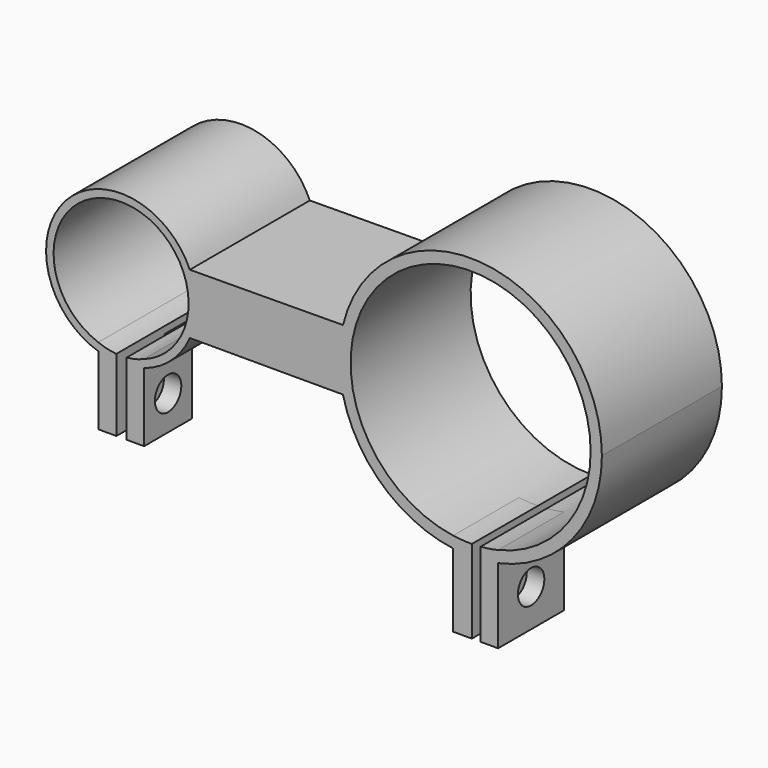
from build123d import *

# Parameters (mm, degrees)
F0_R      = 12.7
F0_R_2    = 11.43
F1_DEPTH  = 25.4
F3_R      = 20.32
F4_DEPTH  = 25.4
F5_W      = 3.0645749275
F5_H      = 25.4
F6_DEPTH  = 10.16
F8_DEPTH  = 30.226
F9_DEPTH  = 25.4
F10_R     = 2.794
F11_DEPTH = 25.4
F13_W     = 3.175
F13_H     = 35.56
F14_DEPTH = 13.97
F15_R     = 2.794
F16_DEPTH = 25.4
F18_DEPTH = 30.734
F20_DEPTH = 40.64
F22_DEPTH = 25.4


with BuildPart() as f1:
    # F0 (on Front) → F1 (new body)
    with BuildSketch(Plane.XZ):
        Circle(F0_R)
        Circle(F0_R_2, mode=Mode.SUBTRACT)
    extrude(amount=F1_DEPTH)

    # F5 (on offset) → F6 (join)
    with BuildSketch(Plane.XZ.offset(25.4)):
        with Locations((-2.327306883, -11.0291545425)):
            Rectangle(F5_W, F5_H)
        Polygon((3.894138498, 1.6708454575), (0.9391864802, 1.6708454575), (0.9391864802, -23.7291545425), (3.894138498, -23.7291545425), (3.894138498, -11.0291545425), align=None)
    extrude(amount=-F6_DEPTH)

    # F7 (on face) → F8 (cut)
    with BuildSketch(Plane.XZ.offset(25.4)):
        Polygon((-3.8595943467, 6.5400209701), (-3.8595943467, -10.7586445001), (-0.7950194192, -10.7537217399), (0.9391864802, -10.7509360094), (3.894138498, -10.7461893413), (3.894138498, 6.8227690223), align=None)
        Polygon((0.9391864802, -10.7509360094), (-0.7950194192, -10.7537217399), (-0.7950194192, -12.6750914838), (0.9391864802, -12.6652251759), (0.9391864802, -11.3913488558), align=None)
    extrude(amount=-F8_DEPTH, mode=Mode.SUBTRACT)

    # F7 (on face) → F9 (cut)
    with BuildSketch(Plane.XZ.offset(25.4)):
        Polygon((-3.8595943467, 6.5400209701), (-3.8595943467, -10.7586445001), (-0.7950194192, -10.7537217399), (0.9391864802, -10.7509360094), (3.894138498, -10.7461893413), (3.894138498, 6.8227690223), align=None)
        Polygon((0.9391864802, -10.7509360094), (-0.7950194192, -10.7537217399), (-0.7950194192, -12.6750914838), (0.9391864802, -12.6652251759), (0.9391864802, -11.3913488558), align=None)
    extrude(amount=-F9_DEPTH, mode=Mode.SUBTRACT)

    # F10 (on face) → F11 (cut)
    with BuildSketch(Plane(origin=(-3.8595943467, 0, 0), x_dir=(0, -1, 0), z_dir=(-1, 0, 0))):
        with Locations((20.32, -17.914237003)):
            Circle(F10_R)
    extrude(amount=-F11_DEPTH, mode=Mode.SUBTRACT)


with BuildPart() as f4:
    # F3 (on offset) → F4 (new body)
    with BuildSketch(Plane.XZ.offset(25.4)):
        with BuildLine():
            Line((37.5699403561, 5.2842361421), (10.6034887032, 5.0843427817))
            ThreePointArc((10.6034887032, 5.0843427817), (11.5328465432, 2.6263680661), (11.8205691299, 0.0143647333))
            Line((11.8205691299, 0.0143647333), (36.950101903, 0.0449029444))
            ThreePointArc((36.950101903, 0.0449029444), (37.1040026209, 2.6830272873), (37.5699403561, 5.2842361421))
        make_face()
        with BuildLine():
            ThreePointArc((81.4000854922, 0.0719114545), (61.799611578, 22.1414036966), (37.5699403561, 5.2842361421))
            Line((37.5699403561, 5.2842361421), (38.7200076161, 5.2927612092))
            ThreePointArc((38.7200076161, 5.2927612092), (37.3247254516, 0.1119146147), (38.6803581082, -5.079447813))
            Line((38.6803581082, -5.079447813), (37.5553231739, -5.079447813))
            ThreePointArc((37.5553231739, -5.079447813), (61.7684816706, -22.0012605256), (81.4000854922, 0.0719114545))
        make_face()
        with Locations((59.1750854922, 0.0719114545)):
            Circle(F3_R, mode=Mode.SUBTRACT)
        with BuildLine():
            Line((38.7200076161, 5.2927612092), (37.5699403561, 5.2842361421))
            ThreePointArc((37.5699403561, 5.2842361421), (37.1040026209, 2.6830272873), (36.950101903, 0.0449029444))
            ThreePointArc((36.950101903, 0.0449029444), (37.1034933748, -2.5348962497), (37.5553231739, -5.079447813))
            Line((37.5553231739, -5.079447813), (38.6803581082, -5.079447813))
            ThreePointArc((38.6803581082, -5.079447813), (37.3247254516, 0.1119146147), (38.7200076161, 5.2927612092))
        make_face()
        with BuildLine():
            Line((36.950101903, 0.0449029444), (11.8205691299, 0.0143647333))
            ThreePointArc((11.8205691299, 0.0143647333), (11.4383828548, -2.6236056978), (10.4021426077, -5.079447813))
            Line((10.4021426077, -5.079447813), (37.5553231739, -5.079447813))
            ThreePointArc((37.5553231739, -5.079447813), (37.1034933748, -2.5348962497), (36.950101903, 0.0449029444))
        make_face()
    extrude(amount=-F4_DEPTH)


with BuildPart() as f1_1:
    add(f1.part)

    # F12: union F4
    add(f4.part)

    # F13 (on face) → F14 (join)
    with BuildSketch(Plane.XZ.offset(25.4)):
        Polygon((63.8311807601, 1.2001052282), (60.8582296082, 1.2001052282), (60.8582296082, -34.3598947718), (63.8311807601, -34.3598947718), (63.8311807601, -21.6598947718), align=None)
        with Locations((57.7986807601, -16.5798947718)):
            Rectangle(F13_W, F13_H)
    extrude(amount=-F14_DEPTH)

    # F15 (on face) → F16 (cut)
    with BuildSketch(Plane.YZ.offset(63.8311807601)):
        with Locations((-18.415, -28.0098947718)):
            Circle(F15_R)
    extrude(amount=-F16_DEPTH, mode=Mode.SUBTRACT)

    # F17 (on face) → F18 (cut)
    with BuildSketch(Plane.XZ.offset(25.4)):
        with BuildLine():
            ThreePointArc((63.8311807601, -19.7074509431), (58.3136851955, 20.3736451127), (56.2111807601, -20.0307666939))
            Line((56.2111807601, -20.0307666939), (56.2111807601, 1.2001052282))
            Line((56.2111807601, 1.2001052282), (59.3861807601, 1.2001052282))
            Line((59.3861807601, 1.2001052282), (60.8582296082, 1.2001052282))
            Line((60.8582296082, 1.2001052282), (63.8311807601, 1.2001052282))
            Line((63.8311807601, 1.2001052282), (63.8311807601, -19.7074509431))
        make_face()
        with BuildLine():
            Line((56.2111807601, 1.2001052282), (56.2111807601, -20.0307666939))
            ThreePointArc((56.2111807601, -20.0307666939), (57.7944413181, -20.2011302922), (59.3861807601, -20.2469920294))
            Line((59.3861807601, -20.2469920294), (59.3861807601, 1.2001052282))
            Line((59.3861807601, 1.2001052282), (56.2111807601, 1.2001052282))
        make_face()
        with BuildLine():
            ThreePointArc((60.8582296082, -20.1782595543), (62.3534347774, -19.9979788248), (63.8311807601, -19.7074509431))
            Line((63.8311807601, -19.7074509431), (63.8311807601, 1.2001052282))
            Line((63.8311807601, 1.2001052282), (60.8582296082, 1.2001052282))
            Line((60.8582296082, 1.2001052282), (60.8582296082, -20.1782595543))
        make_face()
        with BuildLine():
            ThreePointArc((60.8582296082, -20.1782595543), (60.1228284685, -20.2259747224), (59.3861807601, -20.2469920294))
            Line((59.3861807601, -20.2469920294), (59.3861807601, -22.1520860209))
            Line((59.3861807601, -22.1520860209), (60.8582296082, -22.0892629477))
            Line((60.8582296082, -22.0892629477), (60.8582296082, -20.1782595543))
        make_face()
        with BuildLine():
            Line((59.3861807601, 1.2001052282), (59.3861807601, -20.2469920294))
            ThreePointArc((59.3861807601, -20.2469920294), (60.1228284685, -20.2259747224), (60.8582296082, -20.1782595543))
            Line((60.8582296082, -20.1782595543), (60.8582296082, 1.2001052282))
            Line((60.8582296082, 1.2001052282), (59.3861807601, 1.2001052282))
        make_face()
        Polygon((60.8582296082, -22.0892629477), (59.3861807601, -22.1520860209), (59.3861807601, -22.3753936589), (60.8582296082, -22.3753936589), align=None)
    extrude(amount=-F18_DEPTH, mode=Mode.SUBTRACT)

    # F19 (on face) → F20 (cut)
    with BuildSketch(Plane.XZ.offset(25.4)):
        with BuildLine():
            Line((-3.8612207101, -9.7461815458), (-3.8595943467, -10.7586445001))
            ThreePointArc((-3.8595943467, -10.7586445001), (0.0185050029, -11.5199534125), (3.894138498, -10.7461893413))
            Line((3.894138498, -10.7461893413), (3.894138498, -9.7337237745))
            Line((3.894138498, -9.7337237745), (-3.8612207101, -9.7461815458))
        make_face()
    extrude(amount=-F20_DEPTH, mode=Mode.SUBTRACT)

    # F21 (on face) → F22 (cut)
    with BuildSketch(Plane.XZ.offset(25.4)):
        Polygon((0.9391864802, -11.4767284574), (-0.7950194192, -11.4886898794), (-0.7950194192, -13.0471941084), (0.9391864802, -13.0471941084), align=None)
    extrude(amount=-F22_DEPTH, mode=Mode.SUBTRACT)


solid = f1_1.part
